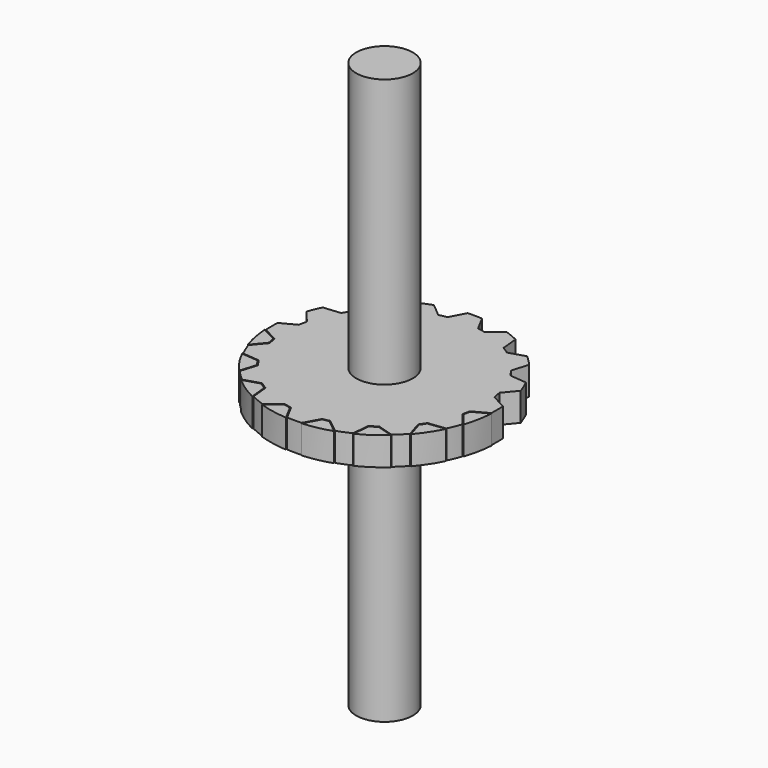
from build123d import *

# Parameters (mm, degrees)
F0_R     = 5
F1_DEPTH = 50
F2_DEPTH = 2.5
F3_DEPTH = 2.5


# Not quite as in the source:
# - a feature names something its author has since deleted; it is built from what else it names
# - the program builds the solid bodies; features that only make, move or delete a surface that nothing else refers to are left out


with BuildPart() as f1:
    # F0 (on Top) → F1 (new body, symmetric)
    with BuildSketch(Plane.XY):
        with Locations((0, -93.1816846132)):
            Circle(F0_R)
    extrude(amount=F1_DEPTH, both=True)


with BuildPart() as f2:
    # F0 (on Top) → F2 (new body, symmetric)
    with BuildSketch(Plane.XY):
        with BuildLine():
            Line((-4.1026274762, -76.169381777), (-6.4206619181, -74.2403250914))
            ThreePointArc((-6.4206619181, -74.2403250914), (-7.6258193304, -74.6925829709), (-8.7993878999, -75.2214292535))
            Line((-8.7993878999, -75.2214292535), (-9.0834852771, -78.2237337101))
            ThreePointArc((-9.0834852771, -78.2237337101), (-9.7042014816, -78.6187702893), (-10.307764064, -79.0395489895))
            Line((-10.307764064, -79.0395489895), (-13.1880158888, -78.1458528465))
            ThreePointArc((-13.1880158888, -78.1458528465), (-14.1421356237, -79.0395489895), (-15.0358317667, -79.9936687244))
            Line((-15.0358317667, -79.9936687244), (-14.1421356237, -82.8739205492))
            ThreePointArc((-14.1421356237, -82.8739205492), (-14.5629143239, -83.4774831316), (-14.9579509031, -84.0981993361))
            Line((-14.9579509031, -84.0981993361), (-17.9602553597, -84.3822967133))
            ThreePointArc((-17.9602553597, -84.3822967133), (-18.4891016423, -85.5558652828), (-18.9413595218, -86.7610226951))
            Line((-18.9413595218, -86.7610226951), (-17.0123028362, -89.079057137))
            ThreePointArc((-17.0123028362, -89.079057137), (-17.1663095757, -89.7805354617), (-17.2914046111, -90.4877420425))
            Line((-17.2914046111, -90.4877420425), (-19.9585764606, -91.8951288747))
            Line((-19.9585764606, -91.8951288747), (-19.9585764606, -93.1816846132))
            Line((-19.9585764606, -93.1816846132), (-19.9585764606, -94.4682403517))
            Line((-19.9585764606, -94.4682403517), (-17.2914046111, -95.875627184))
            ThreePointArc((-17.2914046111, -95.875627184), (-17.1663095757, -96.5828337648), (-17.0123028362, -97.2843120894))
            Line((-17.0123028362, -97.2843120894), (-18.9413595218, -99.6023465313))
            ThreePointArc((-18.9413595218, -99.6023465313), (-18.4891016423, -100.8075039436), (-17.9602553597, -101.9810725131))
            Line((-17.9602553597, -101.9810725131), (-14.9685630672, -102.2476715812))
            ThreePointArc((-14.9685630672, -102.2476715812), (-14.5629143239, -102.8858860948), (-14.1300718682, -103.5059796981))
            Line((-14.1300718682, -103.5059796981), (-15.0358317667, -106.369700502))
            ThreePointArc((-15.0358317667, -106.369700502), (-14.1563340221, -107.3096075693), (-13.2181957315, -108.1909917793))
            Line((-13.2181957315, -108.1909917793), (-10.336154315, -107.3030837641))
            ThreePointArc((-10.336154315, -107.3030837641), (-9.7294103647, -107.727769102), (-9.1052409735, -108.1264023026))
            Line((-9.1052409735, -108.1264023026), (-8.7993878999, -111.141939973))
            ThreePointArc((-8.7993878999, -111.141939973), (-7.6258193304, -111.6707862556), (-6.4206619181, -112.123044135))
            Line((-6.4206619181, -112.123044135), (-4.1026274762, -110.1939874495))
            ThreePointArc((-4.1026274762, -110.1939874495), (-3.3914061607, -110.3499216879), (-2.6743139613, -110.4761358863))
            Line((-2.6743139613, -110.4761358863), (-1.2464570661, -113.142805443))
            ThreePointArc((-1.2464570661, -113.142805443), (0.0401792946, -113.1816442538), (1.3266492185, -113.1376361528))
            Line((1.3266492185, -113.1376361528), (2.8086979778, -110.4548202773))
            ThreePointArc((2.8086979778, -110.4548202773), (3.4183906996, -110.3445691326), (4.0237985116, -110.2128045276))
            Line((4.0237985116, -110.2128045276), (6.4206619181, -112.123044135))
            ThreePointArc((6.4206619181, -112.123044135), (7.6258193304, -111.6707862556), (8.7993878999, -111.141939973))
            Line((8.7993878999, -111.141939973), (9.0834852771, -108.1396355164))
            ThreePointArc((9.0834852771, -108.1396355164), (9.7291988524, -107.7279105736), (10.3562811803, -107.2883298599))
            Line((10.3562811803, -107.2883298599), (13.2483222263, -108.1644066019))
            ThreePointArc((13.2483222263, -108.1644066019), (14.184687954, -107.2811394838), (15.0622956837, -106.3394674332))
            Line((15.0622956837, -106.3394674332), (14.1628150198, -103.4610168248))
            ThreePointArc((14.1628150198, -103.4610168248), (14.5487834975, -102.9070585774), (14.9130966677, -102.3386244831))
            Line((14.9130966677, -102.3386244831), (17.9602553597, -101.9810725131))
            ThreePointArc((17.9602553597, -101.9810725131), (18.4891016423, -100.8075039436), (18.9413595218, -99.6023465313))
            Line((18.9413595218, -99.6023465313), (17.0182547654, -97.259552284))
            ThreePointArc((17.0182547654, -97.259552284), (17.1628845194, -96.6000753129), (17.2819687479, -95.9355103516))
            Line((17.2819687479, -95.9355103516), (19.9559515396, -94.5083338317))
            Line((19.9559515396, -94.5083338317), (19.9585361847, -93.2217806894))
            Line((19.9585361847, -93.2217806894), (19.9611208298, -91.9352275472))
            Line((19.9611208298, -91.9352275472), (17.2967817532, -90.5224853008))
            ThreePointArc((17.2967817532, -90.5224853008), (17.1697173115, -89.7977804415), (17.0123028362, -89.079057137))
            Line((17.0123028362, -89.079057137), (18.9413595218, -86.7610226951))
            ThreePointArc((18.9413595218, -86.7610226951), (18.4891016423, -85.5558652828), (17.9602553597, -84.3822967133))
            Line((17.9602553597, -84.3822967133), (14.9579509031, -84.0981993361))
            ThreePointArc((14.9579509031, -84.0981993361), (14.5531592728, -83.4628598293), (14.1213991508, -82.8455302983))
            Line((14.1213991508, -82.8455302983), (15.009307166, -79.9634888818))
            ThreePointArc((15.009307166, -79.9634888818), (14.1279229561, -79.0253505911), (13.1880158888, -78.1458528465))
            Line((13.1880158888, -78.1458528465), (10.307764064, -79.0395489895))
            ThreePointArc((10.307764064, -79.0395489895), (9.7042014816, -78.6187702893), (9.0834852771, -78.2237337101))
            Line((9.0834852771, -78.2237337101), (8.7993878999, -75.2214292535))
            ThreePointArc((8.7993878999, -75.2214292535), (7.6258193304, -74.6925829709), (6.4206619181, -74.2403250914))
            Line((6.4206619181, -74.2403250914), (4.1026274762, -76.169381777))
            ThreePointArc((4.1026274762, -76.169381777), (3.4011491515, -76.0153750375), (2.6939425707, -75.8902800021))
            Line((2.6939425707, -75.8902800021), (1.2865557385, -73.2231081527))
            ThreePointArc((1.2865557385, -73.2231081527), (0.6436112138, -73.1920431806), (0, -73.1816846132))
            ThreePointArc((0, -73.1816846132), (-0.6436112138, -73.1920431806), (-1.2865557385, -73.2231081527))
            Line((-1.2865557385, -73.2231081527), (-2.6939425707, -75.8902800021))
            ThreePointArc((-2.6939425707, -75.8902800021), (-3.4011491515, -76.0153750375), (-4.1026274762, -76.169381777))
        make_face()
        with Locations((0, -93.1816846132)):
            Circle(F0_R, mode=Mode.SUBTRACT)
    extrude(amount=F2_DEPTH, both=True)


with BuildPart() as f3:
    # F0 (on Top) → F3 (new body, symmetric)
    with BuildSketch(Plane.XY):
        with BuildLine():
            Line((-17.4278441118, -95.9732339822), (-20.0625118464, -94.5829985995))
            ThreePointArc((-20.0625118464, -94.5829985995), (-19.7321928289, -97.0946799783), (-19.0886980781, -99.5448980313))
            Line((-19.0886980781, -99.5448980313), (-18.8839318475, -99.2988424443))
            Line((-18.8839318475, -99.2988424443), (-17.1756516165, -97.2461021379))
            ThreePointArc((-17.1756516165, -97.2461021379), (-17.3134493239, -96.6119864622), (-17.4278441118, -95.9732339822))
        make_face()
    extrude(amount=F3_DEPTH, both=True)


with BuildPart() as f3b:
    # F0 (on Top) → F3, piece 2 (new body, symmetric)
    with BuildSketch(Plane.XY):
        with BuildLine():
            ThreePointArc((19.0885160571, -99.5452025325), (19.7282098357, -97.1145083808), (20.0596771358, -94.6230004803))
            Line((20.0596771358, -94.6230004803), (19.7864465315, -94.768831001))
            Line((19.7864465315, -94.768831001), (17.418193425, -96.0328313668))
            ThreePointArc((17.418193425, -96.0328313668), (17.3099949581, -96.6293758046), (17.1813720516, -97.2218522365))
            Line((17.1813720516, -97.2218522365), (18.8845987244, -99.2967832239))
            Line((18.8845987244, -99.2967832239), (19.0885160571, -99.5452025325))
        make_face()
    extrude(amount=F3_DEPTH, both=True)


with BuildPart() as f3c:
    # F0 (on Top) → F3, piece 3 (new body, symmetric)
    with BuildSketch(Plane.XY):
        with BuildLine():
            Line((8.9741585505, -110.8872480979), (8.941409351, -111.2333374159))
            ThreePointArc((8.941409351, -111.2333374159), (11.2014087876, -109.9218538699), (13.2722702295, -108.3283924071))
            Line((13.2722702295, -108.3283924071), (12.9455754835, -108.2294278128))
            Line((12.9455754835, -108.2294278128), (10.3843919739, -107.4535766859))
            ThreePointArc((10.3843919739, -107.4535766859), (9.8127203562, -107.8525066492), (9.2257415735, -108.2285511448))
            Line((9.2257415735, -108.2285511448), (8.9741585505, -110.8872480979))
        make_face()
    extrude(amount=F3_DEPTH, both=True)


with BuildPart() as f3d:
    # F0 (on Top) → F3, piece 4 (new body, symmetric)
    with BuildSketch(Plane.XY):
        with BuildLine():
            Line((1.5918630958, -112.9677522338), (1.4190830131, -113.2805200467))
            ThreePointArc((1.4190830131, -113.2805200467), (3.934981449, -112.9418804335), (6.3881653122, -112.2889557361))
            Line((6.3881653122, -112.2889557361), (6.110596669, -112.0677405368))
            Line((6.110596669, -112.0677405368), (3.9871793865, -110.375430585))
            ThreePointArc((3.9871793865, -110.375430585), (3.4476911913, -110.4916795713), (2.9048323458, -110.5910053651))
            Line((2.9048323458, -110.5910053651), (1.5918630958, -112.9677522338))
        make_face()
    extrude(amount=F3_DEPTH, both=True)


with BuildPart() as f3e:
    # F0 (on Top) → F3, piece 5 (new body, symmetric)
    with BuildSketch(Plane.XY):
        with BuildLine():
            ThreePointArc((15.225181808, -106.3578138581), (16.7622505287, -104.3297570431), (18.0308773002, -102.1238148835))
            Line((18.0308773002, -102.1238148835), (17.7022509045, -102.1623757288))
            Line((17.7022509045, -102.1623757288), (15.0026577234, -102.4791445477))
            ThreePointArc((15.0026577234, -102.4791445477), (14.6741973125, -102.9893567751), (14.3283927934, -103.487976864))
            Line((14.3283927934, -103.487976864), (15.1249297653, -106.0369947843))
            Line((15.1249297653, -106.0369947843), (15.225181808, -106.3578138581))
        make_face()
    extrude(amount=F3_DEPTH, both=True)


with BuildPart() as f3f:
    # F0 (on Top) → F3, piece 6 (new body, symmetric)
    with BuildSketch(Plane.XY):
        with BuildLine():
            Line((-6.1171577311, -112.0656164414), (-6.3863106942, -112.2896041931))
            ThreePointArc((-6.3863106942, -112.2896041931), (-3.8951209972, -112.9498086087), (-1.3399510633, -113.2859671804))
            Line((-1.3399510633, -113.2859671804), (-1.5067708222, -112.9744141291))
            Line((-1.5067708222, -112.9744141291), (-2.771309172, -110.6127587475))
            ThreePointArc((-2.771309172, -110.6127587475), (-3.4202485266, -110.497122812), (-4.0644175121, -110.3573362832))
            Line((-4.0644175121, -110.3573362832), (-6.1171577311, -112.0656164414))
        make_face()
    extrude(amount=F3_DEPTH, both=True)


with BuildPart() as f3g:
    # F0 (on Top) → F3, piece 7 (new body, symmetric)
    with BuildSketch(Plane.XY):
        with BuildLine():
            Line((-12.9159771829, -108.2548406666), (-13.2417652424, -108.355210435))
            ThreePointArc((-13.2417652424, -108.355210435), (-11.1842983703, -109.9333723769), (-8.9408554374, -111.2336526744))
            Line((-8.9408554374, -111.2336526744), (-8.9760890259, -110.8862694939))
            Line((-8.9760890259, -110.8862694939), (-9.2469724028, -108.2155131802))
            ThreePointArc((-9.2469724028, -108.2155131802), (-9.8124861535, -107.8526632952), (-10.363779415, -107.4685518779))
            Line((-10.363779415, -107.4685518779), (-12.9159771829, -108.2548406666))
        make_face()
    extrude(amount=F3_DEPTH, both=True)


with BuildPart() as f3h:
    # F0 (on Top) → F3, piece 8 (new body, symmetric)
    with BuildSketch(Plane.XY):
        with BuildLine():
            Line((-17.7063489474, -102.1542933171), (-18.0301571677, -102.1254377527))
            ThreePointArc((-18.0301571677, -102.1254377527), (-16.7507329053, -104.3472406327), (-15.1990035025, -106.3881890254))
            Line((-15.1990035025, -106.3881890254), (-15.0979454061, -106.0686759034))
            Line((-15.0979454061, -106.0686759034), (-14.2959294395, -103.5329599675))
            ThreePointArc((-14.2959294395, -103.5329599675), (-14.6877393038, -102.9690649647), (-15.0573191219, -102.3903566598))
            Line((-15.0573191219, -102.3903566598), (-17.7063489474, -102.1542933171))
        make_face()
    extrude(amount=F3_DEPTH, both=True)


solid = Compound([f1.part, f2.part, f3.part, f3b.part, f3c.part, f3d.part, f3e.part, f3f.part, f3g.part, f3h.part])
